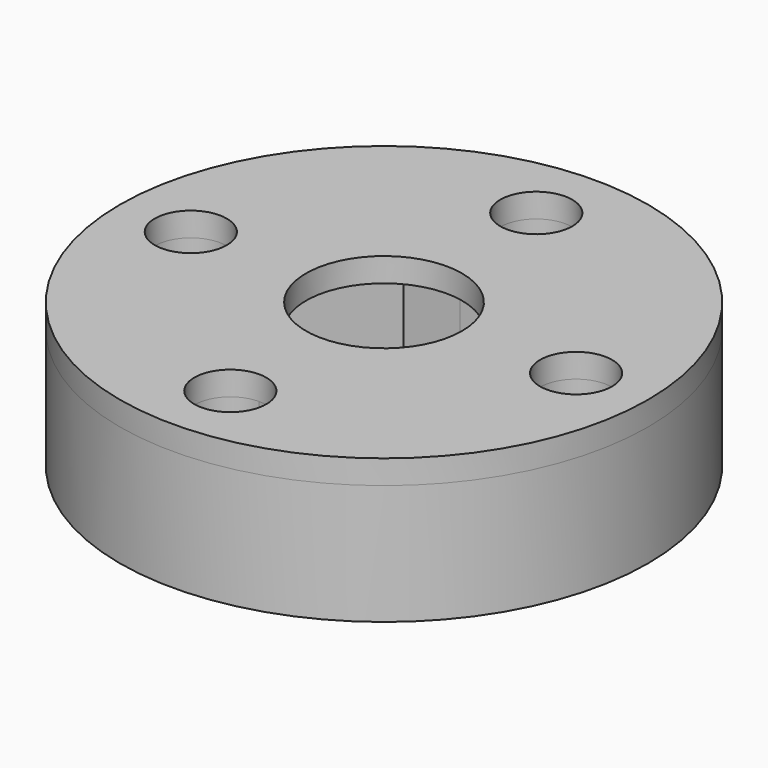
from build123d import *
from build123d import SkipClean  # not in build123d's __all__

# Parameters (mm, degrees)
F0_R     = 11
F1_DEPTH = 5
F2_R     = 11
F2_R_2   = 1.5
F2_R_3   = 3.25
F3_DEPTH = 1


with BuildPart() as f1:
    # F0 (on Top) → F1 (new body)
    with BuildSketch(Plane.XY):
        Circle(F0_R)
        with BuildLine():
            ThreePointArc((-6.4997900966, -0.0579517981), (-9.4997802573, -0.0633848148), (-6.4998294535, -0.0470858359))
            ThreePointArc((-6.4998294535, -0.0470858359), (-6.4997999358, -0.0525187813), (-6.4997900966, -0.0579517981))
        make_face(mode=Mode.SUBTRACT)
        with BuildLine():
            ThreePointArc((1.5, -8), (-1.0606601718, -9.0606601718), (0, -6.5))
            ThreePointArc((0, -6.5), (1.0606601718, -6.9393398282), (1.5, -8))
        make_face(mode=Mode.SUBTRACT)
        with BuildLine():
            ThreePointArc((1.4420482019, 7.9997900966), (1.0065431393, 6.9429786051), (-0.0470858359, 6.4998294535))
            ThreePointArc((-0.0470858359, 6.4998294535), (-1.1224467354, 9.056601588), (1.4420482019, 7.9997900966))
        make_face(mode=Mode.SUBTRACT)
        Polygon((-0.0289763065, 3.9999512958), (2.259031561, 4.0286610356), (4.6184385806, 0.0579517981), (4.5859426869, 0), (2.3594070196, -3.9707092376), (0, -4.0003148882), (-2.259031561, -4.0286610356), (-4.6184385806, -0.0579517981), (-4.6046471933, -0.0333568232), (-2.3594070196, 3.9707092376), align=None, mode=Mode.SUBTRACT)
        with BuildLine():
            ThreePointArc((9.5, 0), (8, -1.5), (6.5, 0))
            ThreePointArc((6.5, 0), (8, 1.5), (9.5, 0))
        make_face(mode=Mode.SUBTRACT)
    extrude(amount=F1_DEPTH)

    # F2 (on face) → F3 (join)
    with BuildSketch(Plane.XY.offset(5)):
        Circle(F2_R)
        with Locations((-7.9997900966, -0.0579517981)):
            Circle(F2_R_2, mode=Mode.SUBTRACT)
        with Locations((0, -8)):
            Circle(F2_R_2, mode=Mode.SUBTRACT)
        with Locations((-0.0579517981, 7.9997900966)):
            Circle(F2_R_2, mode=Mode.SUBTRACT)
        Polygon((-4.6184385806, -0.0579517981), (-2.3594070196, 3.9707092376), (2.259031561, 4.0286610356), (4.6184385806, 0.0579517981), (2.3594070196, -3.9707092376), (-2.259031561, -4.0286610356), align=None, mode=Mode.SUBTRACT)
        with Locations((8, 0)):
            Circle(F2_R_2, mode=Mode.SUBTRACT)
        Polygon((2.259031561, 4.0286610356), (-2.3594070196, 3.9707092376), (-4.6184385806, -0.0579517981), (-2.259031561, -4.0286610356), (2.3594070196, -3.9707092376), (4.6184385806, 0.0579517981), align=None)
        Circle(F2_R_3, mode=Mode.SUBTRACT)
    with SkipClean():  # cleaning this boolean's faces spoils the solid; the shape is the same uncleaned
        extrude(amount=F3_DEPTH)


solid = f1.part
